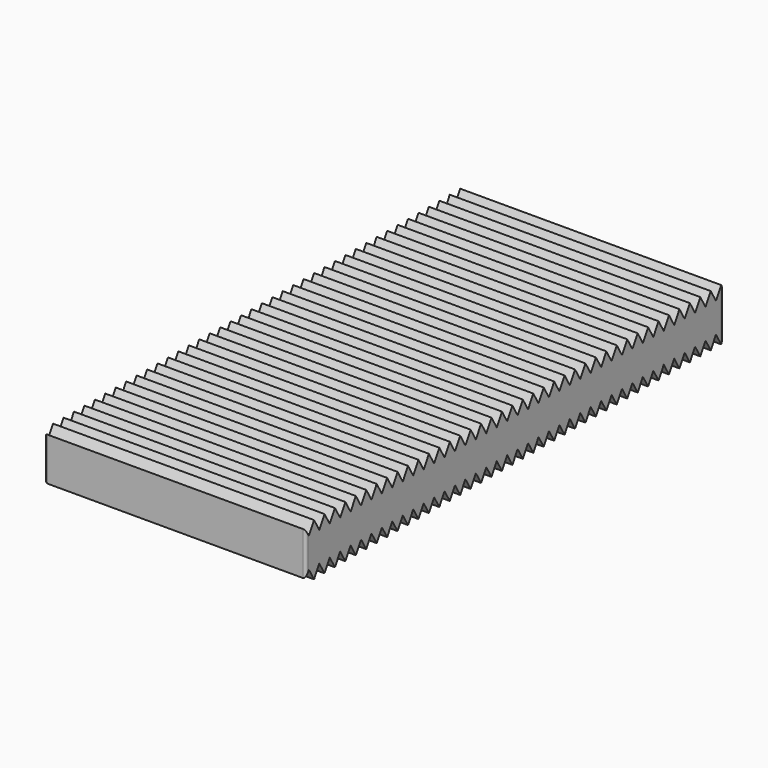
from build123d import *

# Parameters (mm, degrees)
F0_W     = 25.4
F0_H     = 5.08
F1_DEPTH = 25.4
F3_DEPTH = 12.7
F4_R     = 0.25399


# Not quite as in the source:
# - a fillet or chamfer is up to 0.001 mm smaller than in the source, because OpenCascade refuses the exact size


with BuildPart() as f1:
    # F0 (on Front) → F1 (new body, symmetric)
    with BuildSketch(Plane.XZ):
        Rectangle(F0_W, F0_H)
    extrude(amount=F1_DEPTH, both=True)

    # F2 (on Right) → F3 (cut, symmetric)
    with BuildSketch(Plane.YZ):
        Polygon((1.6510001588, -1.4401473588), (1.0160001588, -2.5399996216), (0.3810001588, -1.4401473588), (-0.2539998412, -2.5399996216), (-0.8889998412, -1.4401473588), (-1.5239998412, -2.5399996216), (-2.1589998412, -1.4401473588), (-2.7939998412, -2.5399996216), (-3.4289998412, -1.4401473588), (-4.0639998412, -2.5399996216), (-4.6989998412, -1.4401473588), (-5.3339998412, -2.5399996216), (-5.9689998412, -1.4401473588), (-6.6039998412, -2.5399996216), (-7.2389998412, -1.4401473588), (-7.8739998412, -2.5399996216), (-8.5089998412, -1.4401473588), (-9.1439998412, -2.5399996216), (-9.7789998412, -1.4401473588), (-10.4139998412, -2.5399996216), (-11.0489998412, -1.4401473588), (-11.6839998412, -2.5399996216), (-12.3189998412, -1.4401473588), (-12.9539998412, -2.5399996216), (-13.5889998412, -1.4401473588), (-14.2239998412, -2.5399996216), (-14.8589998412, -1.4401473588), (-15.4939998412, -2.5399996216), (-16.1289998412, -1.4401473588), (-16.7639998412, -2.5399996216), (-17.3989998412, -1.4401473588), (-18.0339998412, -2.5399996216), (-18.6689998412, -1.4401473588), (-19.3039998412, -2.5399996216), (-19.9389998412, -1.4401473588), (-20.5739998412, -2.5399996216), (-21.2089998412, -1.4401473588), (-21.8439998412, -2.5399996216), (-22.4789998412, -1.4401473588), (-23.1139998412, -2.5399996216), (-23.7489998412, -1.4401473588), (-24.3839998412, -2.5399996216), (-25.0189998412, -1.4401473588), (-25.6539998412, -2.5399996216), (-26.2889998412, -1.4401473588), (-26.9239998412, -2.5399996216), (-27.5589998412, -1.4401473588), (-28.1939998412, -2.5399996216), (-28.8289998412, -1.4401473588), (-29.4639998412, -2.5399996216), (-29.4639998412, -2.7939996216), (31.4960001588, -2.7939996216), (31.4960001588, -2.5399996216), (30.8610001588, -1.4401473588), (30.2260001588, -2.5399996216), (29.5910001588, -1.4401473588), (28.9560001588, -2.5399996216), (28.3210001588, -1.4401473588), (27.6860001588, -2.5399996216), (27.0510001588, -1.4401473588), (26.4160001588, -2.5399996216), (25.7810001588, -1.4401473588), (25.1460001588, -2.5399996216), (24.5110001588, -1.4401473588), (23.8760001588, -2.5399996216), (23.2410001588, -1.4401473588), (22.6060001588, -2.5399996216), (21.9710001588, -1.4401473588), (21.3360001588, -2.5399996216), (20.7010001588, -1.4401473588), (20.0660001588, -2.5399996216), (19.4310001588, -1.4401473588), (18.7960001588, -2.5399996216), (18.1610001588, -1.4401473588), (17.5260001588, -2.5399996216), (16.8910001588, -1.4401473588), (16.2560001588, -2.5399996216), (15.6210001588, -1.4401473588), (14.9860001588, -2.5399996216), (14.3510001588, -1.4401473588), (13.7160001588, -2.5399996216), (13.0810001588, -1.4401473588), (12.4460001588, -2.5399996216), (11.8110001588, -1.4401473588), (11.1760001588, -2.5399996216), (10.5410001588, -1.4401473588), (9.9060001588, -2.5399996216), (9.2710001588, -1.4401473588), (8.6360001588, -2.5399996216), (8.0010001588, -1.4401473588), (7.3660001588, -2.5399996216), (6.7310001588, -1.4401473588), (6.0960001588, -2.5399996216), (5.4610001588, -1.4401473588), (4.8260001588, -2.5399996216), (4.1910001588, -1.4401473588), (3.5560001588, -2.5399996216), (2.9210001588, -1.4401473588), (2.2860001588, -2.5399996216), align=None)
        Polygon((31.4960001588, 2.5399996216), (31.4960001588, 2.7939996216), (-29.4639998412, 2.7939996216), (-29.4639998412, 2.5399996216), (-28.8289998412, 1.4401473588), (-28.1939998412, 2.5399996216), (-27.5589998412, 1.4401473588), (-26.9239998412, 2.5399996216), (-26.2889998412, 1.4401473588), (-25.6539998412, 2.5399996216), (-25.0189998412, 1.4401473588), (-24.3839998412, 2.5399996216), (-23.7489998412, 1.4401473588), (-23.1139998412, 2.5399996216), (-22.4789998412, 1.4401473588), (-21.8439998412, 2.5399996216), (-21.2089998412, 1.4401473588), (-20.5739998412, 2.5399996216), (-19.9389998412, 1.4401473588), (-19.3039998412, 2.5399996216), (-18.6689998412, 1.4401473588), (-18.0339998412, 2.5399996216), (-17.3989998412, 1.4401473588), (-16.7639998412, 2.5399996216), (-16.1289998412, 1.4401473588), (-15.4939998412, 2.5399996216), (-14.8589998412, 1.4401473588), (-14.2239998412, 2.5399996216), (-13.5889998412, 1.4401473588), (-12.9539998412, 2.5399996216), (-12.3189998412, 1.4401473588), (-11.6839998412, 2.5399996216), (-11.0489998412, 1.4401473588), (-10.4139998412, 2.5399996216), (-9.7789998412, 1.4401473588), (-9.1439998412, 2.5399996216), (-8.5089998412, 1.4401473588), (-7.8739998412, 2.5399996216), (-7.2389998412, 1.4401473588), (-6.6039998412, 2.5399996216), (-5.9689998412, 1.4401473588), (-5.3339998412, 2.5399996216), (-4.6989998412, 1.4401473588), (-4.0639998412, 2.5399996216), (-3.4289998412, 1.4401473588), (-2.7939998412, 2.5399996216), (-2.1589998412, 1.4401473588), (-1.5239998412, 2.5399996216), (-0.8889998412, 1.4401473588), (-0.2539998412, 2.5399996216), (0.3810001588, 1.4401473588), (1.0160001588, 2.5399996216), (1.6510001588, 1.4401473588), (2.2860001588, 2.5399996216), (2.9210001588, 1.4401473588), (3.5560001588, 2.5399996216), (4.1910001588, 1.4401473588), (4.8260001588, 2.5399996216), (5.4610001588, 1.4401473588), (6.0960001588, 2.5399996216), (6.7310001588, 1.4401473588), (7.3660001588, 2.5399996216), (8.0010001588, 1.4401473588), (8.6360001588, 2.5399996216), (9.2710001588, 1.4401473588), (9.9060001588, 2.5399996216), (10.5410001588, 1.4401473588), (11.1760001588, 2.5399996216), (11.8110001588, 1.4401473588), (12.4460001588, 2.5399996216), (13.0810001588, 1.4401473588), (13.7160001588, 2.5399996216), (14.3510001588, 1.4401473588), (14.9860001588, 2.5399996216), (15.6210001588, 1.4401473588), (16.2560001588, 2.5399996216), (16.8910001588, 1.4401473588), (17.5260001588, 2.5399996216), (18.1610001588, 1.4401473588), (18.7960001588, 2.5399996216), (19.4310001588, 1.4401473588), (20.0660001588, 2.5399996216), (20.7010001588, 1.4401473588), (21.3360001588, 2.5399996216), (21.9710001588, 1.4401473588), (22.6060001588, 2.5399996216), (23.2410001588, 1.4401473588), (23.8760001588, 2.5399996216), (24.5110001588, 1.4401473588), (25.1460001588, 2.5399996216), (25.7810001588, 1.4401473588), (26.4160001588, 2.5399996216), (27.0510001588, 1.4401473588), (27.6860001588, 2.5399996216), (28.3210001588, 1.4401473588), (28.9560001588, 2.5399996216), (29.5910001588, 1.4401473588), (30.2260001588, 2.5399996216), (30.8610001588, 1.4401473588), align=None)
    extrude(amount=F3_DEPTH, both=True, mode=Mode.SUBTRACT)

    # F4 (radius 0.254 in the source; OpenCascade refuses exactly that, so slightly less here)
    f4_edges = [f1.edges().sort_by_distance(p)[0] for p in [
        (12.7, -25.4, 0),
        (-12.7, -25.4, 0),
        (-12.7, 25.4, 0),
        (0, 25.4, 2.100059),
        (12.7, 25.4, 0),
        (0, 25.4, -2.100059),
    ]]
    fillet(f4_edges, radius=F4_R)


solid = f1.part
